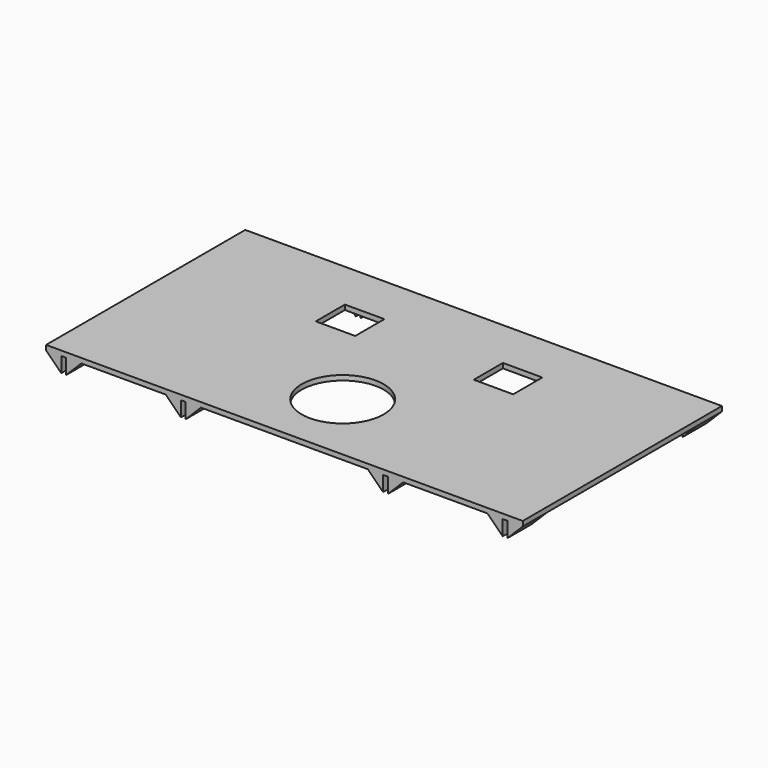
from build123d import *

# Parameters (mm, degrees)
F2_DEPTH  = 82
F3_DEPTH  = 10
F4_START  = -72
F4_DEPTH  = 10
F7_DEPTH  = 10
F8_START  = 102.8
F8_DEPTH  = 10
F10_R     = 13.5
F11_DEPTH = 1.6
F12_W     = 13
F12_H     = 12
F13_DEPTH = 1.6


# Not quite as in the source:
# - a feature names something its author has since deleted; it is built from what else it names


with BuildPart() as f2:
    # F1 (on offset) → F2 (new body)
    with BuildSketch(Plane.XZ.offset(41)):
        Polygon((78.5, 0), (78.5, 1.6), (-78.5, 1.6), (-78.5, 0), (-73.5, 0), (-71.9, 0), (-66.9, 0), (-39.1, 0), (-34.1, 0), (-32.5, 0), (-27.5, 0), (27.5, 0), (32.5, 0), (34.1, 0), (39.1, 0), (66.9, 0), (71.9, 0), (73.5, 0), align=None)
    extrude(amount=-F2_DEPTH)

    # F1 (on offset) → F3 (join)
    with BuildSketch(Plane.XZ.offset(41)):
        Polygon((-66.9, 0), (-71.9, 0), (-71.9, -5), align=None)
        Polygon((-34.1, 0), (-39.1, 0), (-34.1, -5), align=None)
        Polygon((-27.5, 0), (-32.5, 0), (-32.5, -5), align=None)
        Polygon((-73.5, 0), (-78.5, 0), (-73.5, -5), align=None)
    extrude(amount=-F3_DEPTH)

    # F1 (on offset) → F4 (join)
    with BuildSketch(Plane.XZ.offset(41).offset(F4_START)):
        Polygon((-66.9, 0), (-71.9, 0), (-71.9, -5), align=None)
        Polygon((-34.1, 0), (-39.1, 0), (-34.1, -5), align=None)
        Polygon((-27.5, 0), (-32.5, 0), (-32.5, -5), align=None)
        Polygon((-73.5, 0), (-78.5, 0), (-73.5, -5), align=None)
    extrude(amount=-F4_DEPTH)

    # F6 (on offset) → F7 (join)
    with BuildSketch(Plane.YZ.offset(-51.4)):
        Polygon((-11.1, 0), (-11.1, -5), (-6.1, 0), align=None)
        Polygon((-14.3, -5), (-14.3, 0), (-19.3, 0), align=None)
    extrude(amount=-F7_DEPTH)

    # F6 (on offset) → F8 (join)
    with BuildSketch(Plane.YZ.offset(-51.4).offset(F8_START)):
        Polygon((-11.1, 0), (-11.1, -5), (-6.1, 0), align=None)
        Polygon((-14.3, -5), (-14.3, 0), (-19.3, 0), align=None)
    extrude(amount=F8_DEPTH)

    # F9: F2 across plane


with BuildPart() as f2_1:
    add(f2.part)
    add(f2.part.mirror(Plane.YZ))

    # F10 (on face) → F11 (cut)
    with BuildSketch(Plane.XY.offset(1.6)):
        with Locations((0, -17.0082943066)):
            Circle(F10_R)
    extrude(amount=-F11_DEPTH, mode=Mode.SUBTRACT)

    # F12 (on face) → F13 (cut)
    with BuildSketch(Plane.XY.offset(1.6)):
        with Locations((-26.0217403993, 18.549364836)):
            Rectangle(F12_W, F12_H)
        with Locations((26.0217403993, 18.549364836)):
            Rectangle(F12_W, F12_H)
    extrude(amount=-F13_DEPTH, mode=Mode.SUBTRACT)


solid = f2_1.part
